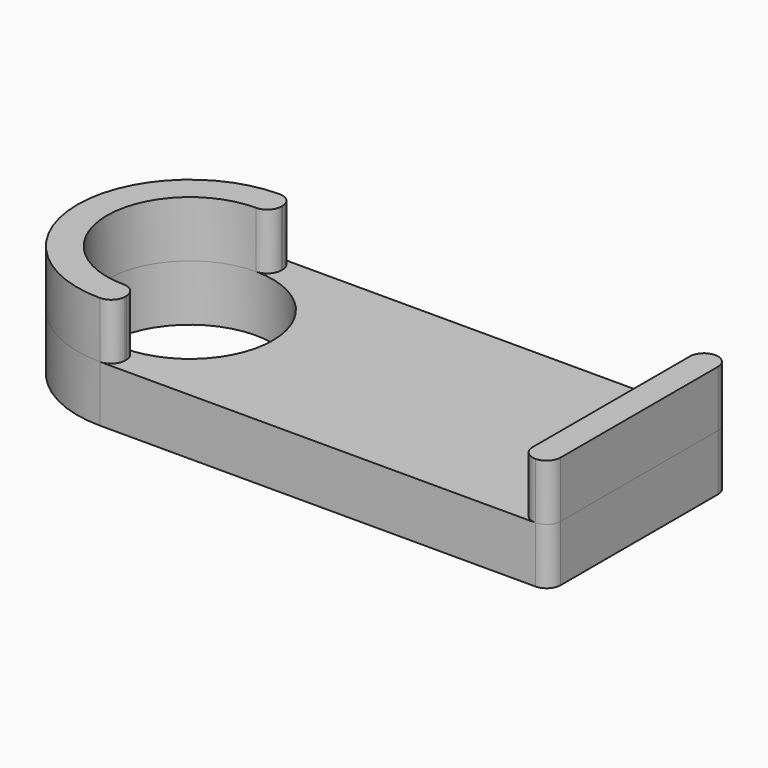
from build123d import *

# Parameters (mm, degrees)
F0_R     = 14.75
F1_DEPTH = 10
F3_DEPTH = 10


# Not quite as in the source:
# - a feature names something its author has since deleted; it is built from what else it names


with BuildPart() as f1:
    # F0 (on Top) → F1 (new body)
    with BuildSketch(Plane.XY):
        with BuildLine():
            ThreePointArc((0, 20), (5.8578643763, 5.8578643763), (20, 0))
            Line((20, 0), (97.5, 0))
            ThreePointArc((97.5, 0), (99.267766953, 0.732233047), (100, 2.5))
            Line((100, 2.5), (100, 37.5))
            ThreePointArc((100, 37.5), (99.267766953, 39.267766953), (97.5, 40))
            Line((97.5, 40), (20, 40))
            ThreePointArc((20, 40), (5.8578643763, 34.1421356237), (0, 20))
        make_face()
        with Locations((20, 20)):
            Circle(F0_R, mode=Mode.SUBTRACT)
    extrude(amount=F1_DEPTH)

    # F2 (on face) → F3 (join)
    with BuildSketch(Plane.XY.offset(10)):
        with BuildLine():
            ThreePointArc((22.5, 37.5), (21.767766953, 39.267766953), (20, 40))
            ThreePointArc((20, 40), (0, 20), (20, 0))
            ThreePointArc((20, 0), (21.767766953, 0.732233047), (22.5, 2.5))
            Line((22.5, 2.5), (22.5, 2.75))
            ThreePointArc((22.5, 2.75), (21.767766953, 4.517766953), (20, 5.25))
            ThreePointArc((20, 5.25), (5.25, 20), (20, 34.75))
            ThreePointArc((20, 34.75), (21.767766953, 35.482233047), (22.5, 37.25))
            Line((22.5, 37.25), (22.5, 37.5))
        make_face()
        with BuildLine():
            ThreePointArc((100, 37.5), (99.267766953, 39.267766953), (97.5, 40))
            ThreePointArc((97.5, 40), (95.732233047, 39.267766953), (95, 37.5))
            Line((95, 37.5), (95, 2.5))
            ThreePointArc((95, 2.5), (95.732233047, 0.732233047), (97.5, 0))
            ThreePointArc((97.5, 0), (99.267766953, 0.732233047), (100, 2.5))
            Line((100, 2.5), (100, 37.5))
        make_face()
    extrude(amount=F3_DEPTH)


solid = f1.part
